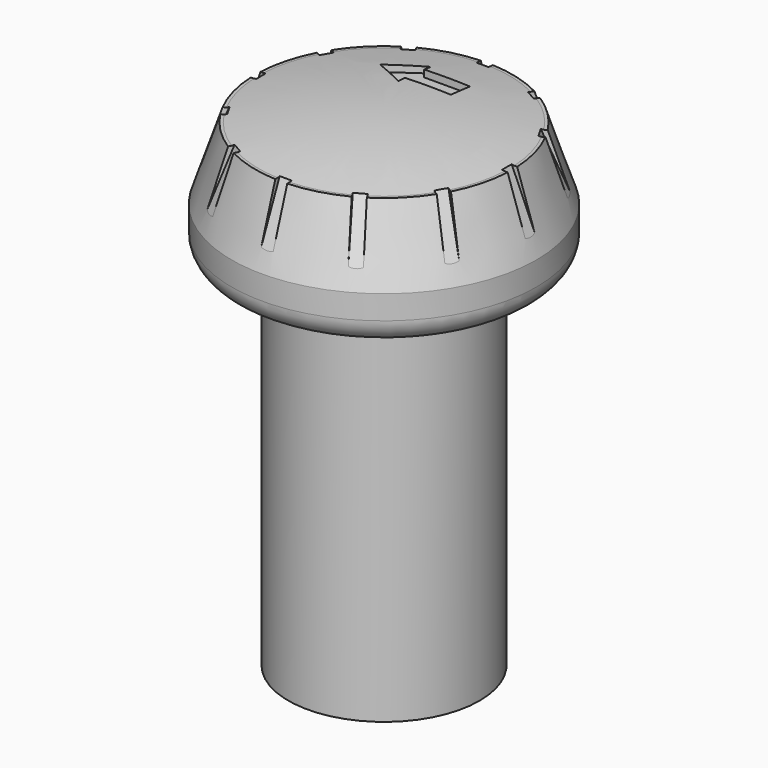
from build123d import *

# Parameters (mm, degrees)
F0_R             = 8
F1_DEPTH         = 30
F2_R             = 12.75
F3_DEPTH         = 10
F4_SIZE2         = 6
F4_SIZE          = 2
F7_R             = 2
F8_R             = 5
F9_DEPTH         = 39
F11_DEPTH        = 28.5
F13_DEPTH        = 0.5
F13_COPIES_COUNT = 12
F15_DEPTH        = 1


# Not quite as in the source:
# - a pattern or mirror of a feature is missing from the dataset's text; its kind, count and spacing are read off the source's solid


with BuildPart() as f1:
    # F0 (on Top) → F1 (new body)
    with BuildSketch(Plane.XY):
        Circle(F0_R)
    extrude(amount=-F1_DEPTH)

    # F2 (on Top) → F3 (join)
    with BuildSketch(Plane.XY):
        Circle(F2_R)
    extrude(amount=F3_DEPTH)

    # F4
    f4_edges = [f1.edges().sort_by_distance(p)[0] for p in [
        (-12.75, 0, 10),
    ]]
    f4_side = f1.faces().sort_by_distance((0, 0, 10))[0]
    chamfer(f4_edges, length=F4_SIZE, length2=F4_SIZE2, reference=f4_side)

    # F5 (on Front) → F6 (revolve)
    with BuildSketch(Plane.XZ):
        with BuildLine():
            Line((0, 10), (10.5, 10))
            ThreePointArc((10.5, 10), (5.2737557774, 10.749435663), (0, 11))
            Line((0, 11), (0, 10))
        make_face()
    revolve(axis=Axis((0, 0, 11.4106573164), (0, 0, -1)))

    # F7
    f7_edges = [f1.edges().sort_by_distance(p)[0] for p in [
        (-12.75, 0, 0),
    ]]
    fillet(f7_edges, radius=F7_R)

    # F8 (on face) → F9 (cut)
    with BuildSketch(Plane(origin=(0, 0, -30), x_dir=(1, 0, 0), z_dir=(0, 0, -1))):
        Circle(F8_R)
    extrude(amount=-F9_DEPTH, mode=Mode.SUBTRACT)

    # F10 (on face) → F11 (join)
    with BuildSketch(Plane(origin=(0, 0, 9), x_dir=(1, 0, 0), z_dir=(0, 0, -1))):
        Polygon((0, 6), (-4.867254519, 3), (5.0389095293, 3), align=None)
    extrude(amount=F11_DEPTH)

    # F12 (on Front) → F13 (cut, symmetric)
    with BuildSketch(Plane.XZ):
        Polygon((-13.3409490809, 2.9869333375), (-9.9859265611, 10.7209142298), (-13.1098602818, 12.8878117818), (-16.7612417104, 4.4706658365), align=None)
    f13 = extrude(amount=F13_DEPTH, both=True, mode=Mode.SUBTRACT)

    # F13_copies: F13 ×12 about axis
    f13_copies_axis = Axis((0, 0, 0), (0, 0, 1))
    for i in range(1, F13_COPIES_COUNT):
        add(f13.rotate(f13_copies_axis, i * 360 / F13_COPIES_COUNT), mode=Mode.SUBTRACT)

    # F14 (on face) → F15 (cut)
    with BuildSketch(Plane.XY.offset(10)):
        Polygon((1.9268689083, 4.5769295732), (1.9268689083, 6.5769295732), (-1.8981318941, 6.5769295732), (-1.8981318941, 7.2769295732), (-4.6231322793, 5.3769295732), (-1.8981318941, 3.8769295732), (-1.8981318941, 4.5769295732), align=None)
    extrude(amount=F15_DEPTH, mode=Mode.SUBTRACT)


solid = f1.part
